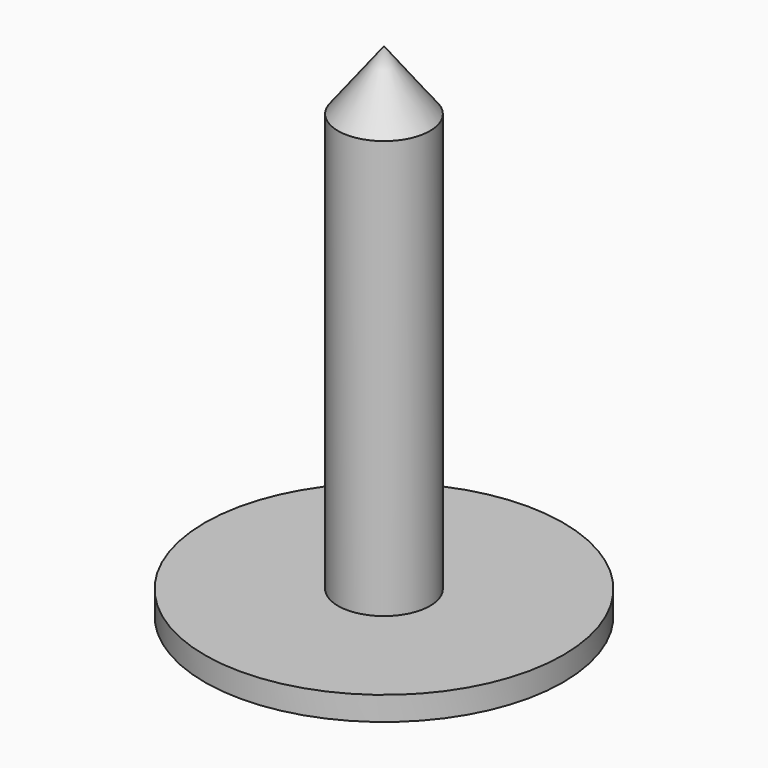
from build123d import *


# Not quite as in the source:
# - a feature names something its author has since deleted; it is built from what else it names


with BuildPart() as f1:
    # F0 (on Front) → F1 (revolve)
    with BuildSketch(Plane.XZ):
        Polygon((0, 53.4480181336), (-3.85, 48.4480181336), (-3.85, 43.4480181336), (-3.85, 33.4480181336), (-3.85, 13.4480181336), (0, 13.4480181336), align=None)
        Polygon((0, 11.4480181336), (0, 13.4480181336), (-3.85, 13.4480181336), (-15, 13.4480181336), (-15, 11.4480181336), align=None)
    revolve(axis=Axis((0, 0, 50.601095613), (0, 0, 1)))


solid = f1.part
